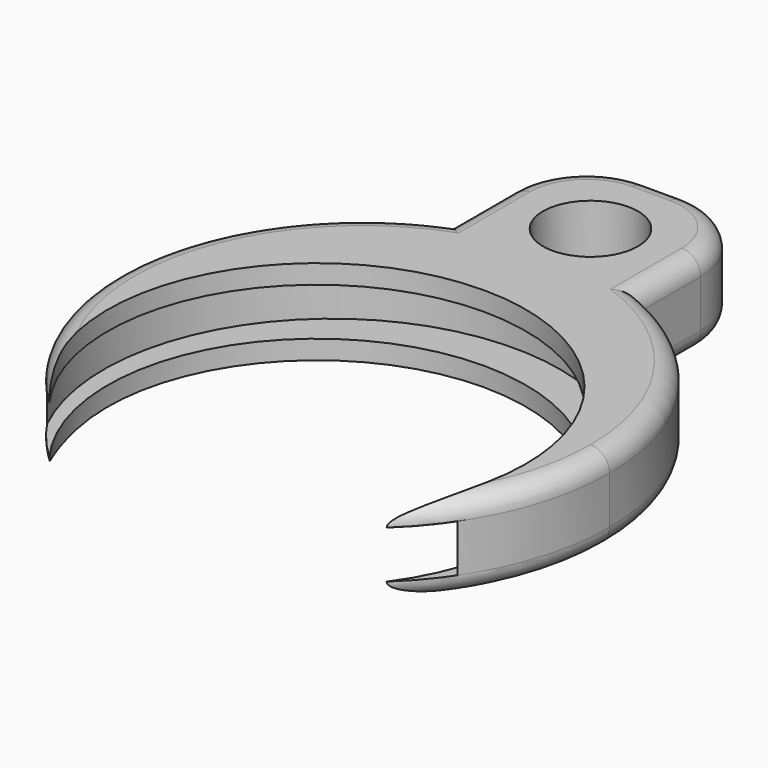
from build123d import *

# Parameters (mm, degrees)
F1_DEPTH  = 4.5
F2_R      = 4
F3_R      = 2.5
F4_DEPTH  = 4.501
F5_R      = 11
F6_DEPTH  = 1
F7_R      = 12
F8_DEPTH  = 2.5
F9_R      = 11
F10_DEPTH = 1.001
F11_R     = 0.99999


# Not quite as in the source:
# - a fillet or chamfer is up to 0.001 mm smaller than in the source, because OpenCascade refuses the exact size


with BuildPart() as f1:
    # F0 (on Top) → F1 (new body)
    with BuildSketch(Plane.XY):
        with BuildLine():
            ThreePointArc((-5, 12), (-7.2111025509, -10.8166538264), (13, 0))
            ThreePointArc((13, 0), (10.8166538264, 7.2111025509), (5, 12))
            Line((5, 12), (-5, 12))
        make_face()
        with BuildLine():
            Line((-5, 12), (5, 12))
            ThreePointArc((5, 12), (0, 13), (-5, 12))
        make_face()
        with BuildLine():
            ThreePointArc((-5, 12), (0, 13), (5, 12))
            Line((5, 12), (5, 20))
            Line((5, 20), (-5, 20))
            Line((-5, 20), (-5, 12))
        make_face()
    extrude(amount=F1_DEPTH)

    # F2
    f2_edges = [f1.edges().sort_by_distance(p)[0] for p in [
        (5, 20, 2.25),
        (-5, 20, 2.25),
    ]]
    fillet(f2_edges, radius=F2_R)

    # F3 (on face) → F4 (cut, through all)
    with BuildSketch(Plane.XY.offset(4.5)):
        with Locations((0, 15)):
            Circle(F3_R)
    extrude(amount=-F4_DEPTH, mode=Mode.SUBTRACT)

    # F5 (on face) → F6 (cut)
    with BuildSketch(Plane.XY.offset(4.5)):
        with Locations((0, -3)):
            Circle(F5_R)
    extrude(amount=-F6_DEPTH, mode=Mode.SUBTRACT)

    # F7 (on face) → F8 (cut)
    with BuildSketch(Plane.XY.offset(3.5)):
        with Locations((0, -2)):
            Circle(F7_R)
    extrude(amount=-F8_DEPTH, mode=Mode.SUBTRACT)

    # F9 (on face) → F10 (cut, through all)
    with BuildSketch(Plane.XY.offset(1)):
        with Locations((0, -3)):
            Circle(F9_R)
    extrude(amount=-F10_DEPTH, mode=Mode.SUBTRACT)

    # F11 (radius 1 in the source; OpenCascade refuses exactly that, so slightly less here)
    f11_edges = [f1.edges().sort_by_distance(p)[0] for p in [
        (12.793956, 2.305363, 4.5),
        (5, 14, 4.5),
        (-12.793956, 2.305363, 4.5),
        (12.793956, 2.305363, 0),
        (-12.793956, 2.305363, 0),
        (-3.828427, 18.828427, 0),
    ]]
    fillet(f11_edges, radius=F11_R)


solid = f1.part
